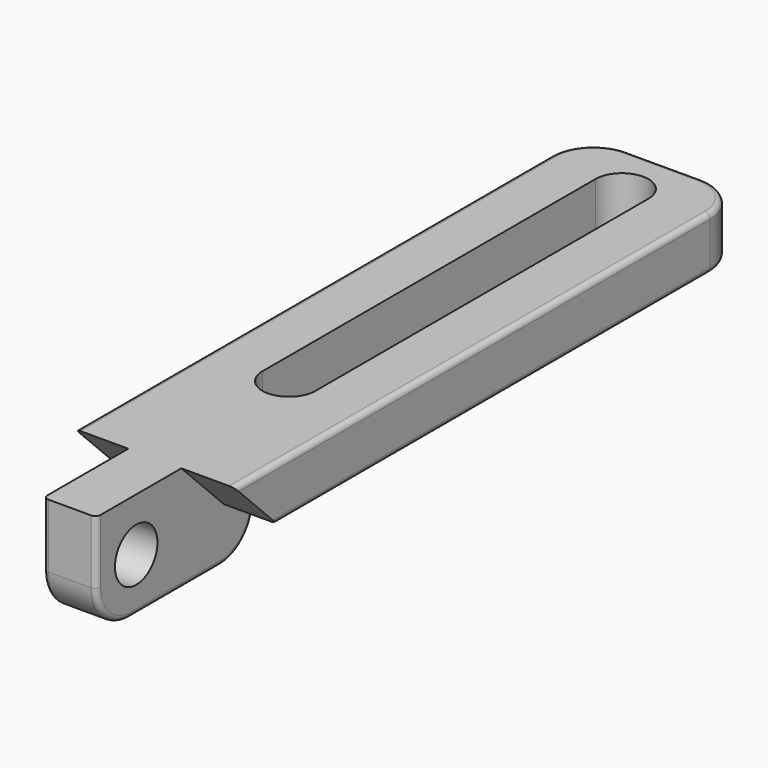
from build123d import *

# Parameters (mm, degrees)
F1_DEPTH = 6.35
F3_DEPTH = 6.35
F5_D     = 6.35
F6_R     = 5.08
F7_R     = 5.08
F8_SIZE  = 6.34999
F9_R     = 5.08
F10_R    = 0.635


# Not quite as in the source:
# - a fillet or chamfer is up to 0.001 mm smaller than in the source, because OpenCascade refuses the exact size
# - a feature names something its author has since deleted; it is built from what else it names


with BuildPart() as f1:
    # F0 (on Top) → F1 (new body)
    with BuildSketch(Plane.XY):
        Polygon((9.525, 38.1), (-9.525, 38.1), (-9.525, -38.1), (-3.175, -38.1), (-3.175, -50.8), (3.175, -50.8), (3.175, -38.1), (9.525, -38.1), align=None)
        with BuildLine():
            ThreePointArc((3.175, -18.0363506079), (0, -21.2113506079), (-3.175, -18.0363506079))
            Line((-3.175, -18.0363506079), (-3.175, 31.75))
            ThreePointArc((-3.175, 31.75), (0, 34.925), (3.175, 31.75))
            Line((3.175, 31.75), (3.175, -18.0363506079))
        make_face(mode=Mode.SUBTRACT)
    extrude(amount=F1_DEPTH)

    # F2 (on face) → F3 (join)
    with BuildSketch(Plane(origin=(0, 0, 0), x_dir=(1, 0, 0), z_dir=(0, 0, -1))):
        Polygon((3.175, 38.1), (3.175, 50.8), (-3.175, 50.8), (-3.175, 38.1), (-3.175, 27.132358402), (3.175, 27.132358402), align=None)
    extrude(amount=F3_DEPTH)

    # F5 (through all)
    with Locations(Plane(origin=(-3.175, 0, 0), x_dir=(0, -1, 0), z_dir=(-1, 0, 0))):
        with Locations((44.8514223099, 0)):
            Hole(F5_D / 2)

    # F6
    f6_edges = [f1.edges().sort_by_distance(p)[0] for p in [
        (0, -50.8, -6.35),
    ]]
    fillet(f6_edges, radius=F6_R)

    # F7
    f7_edges = [f1.edges().sort_by_distance(p)[0] for p in [
        (-9.525, 38.1, 3.175),
        (9.525, 38.1, 3.175),
    ]]
    fillet(f7_edges, radius=F7_R)

    # F8 (size 6.35 in the source; OpenCascade refuses exactly that, so slightly less here)
    f8_edges = [f1.edges().sort_by_distance(p)[0] for p in [
        (6.35, -38.1, 0),
        (-6.35, -38.1, 0),
    ]]
    chamfer(f8_edges, length=F8_SIZE)

    # F9
    f9_edges = [f1.edges().sort_by_distance(p)[0] for p in [
        (0, -27.132358, -6.35),
    ]]
    fillet(f9_edges, radius=F9_R)

    # F10
    f10_edges = [f1.edges().sort_by_distance(p)[0] for p in [
        (-3.175, -50.8, 2.54),
        (3.175, -50.8, 2.54),
        (-9.525, 0.634995, 0),
        (9.525, -2.54, 6.35),
    ]]
    fillet(f10_edges, radius=F10_R)


solid = f1.part
